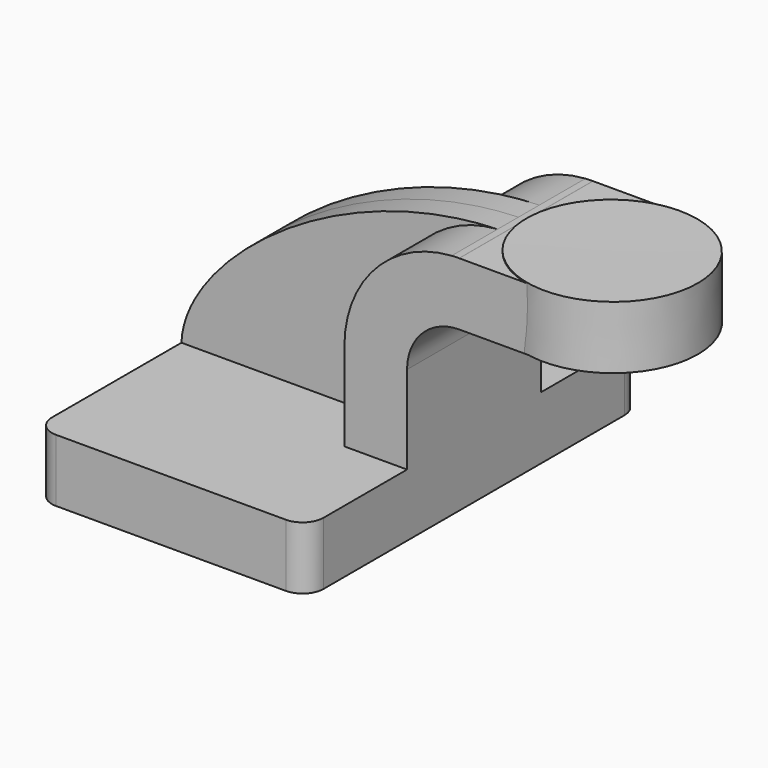
from build123d import *

# Parameters (mm, degrees)
F1_DEPTH = 63.5
F2_DEPTH = 25.4
F3_DEPTH = 7.9375
F5_R     = 6.35


# Not quite as in the source:
# - ends of sketch curves that miss each other by under 0.0002 mm in the source are joined


with BuildPart() as f1:
    # F0 (on Front) → F1 (new body, symmetric)
    with BuildSketch(Plane.XZ):
        Polygon((22.225, 9.525), (-41.275, 9.525), (-41.275, -9.525), (41.275, -9.525), (41.275, 9.525), align=None)
    extrude(amount=F1_DEPTH, both=True)

    # F0 (on Front) → F2 (join, symmetric)
    with BuildSketch(Plane.XZ):
        with BuildLine():
            Line((22.225, 36.2963777006), (22.225, 9.525))
            Line((22.225, 9.525), (41.275, 9.525))
            Line((41.275, 9.525), (41.275, 36.2963777006))
            ThreePointArc((41.275, 36.2963777006), (45.9064737786, 47.5034622059), (57.0984636988, 52.1712940471))
            Line((57.0984636988, 52.1712940471), (57.0984634272, 71.2213777006))
            ThreePointArc((57.0984634272, 71.2213777006), (55.9576218184, 71.2010172098), (54.8180528643, 71.1434385172))
            ThreePointArc((54.8180528643, 71.1434385172), (31.6431491682, 60.1533721811), (22.225, 36.2963777006))
        make_face()
        with BuildLine():
            ThreePointArc((57.15, 71.2213777006), (57.1242317347, 71.2213681944), (57.0984634834, 71.221339676))
            Line((57.0984634834, 71.221339676), (57.0984634272, 52.1713777006))
            ThreePointArc((57.0984634272, 52.1713777006), (57.1242318155, 52.1713567872), (57.15, 52.1713777006))
            Line((57.15, 52.1713777006), (83.1548832357, 52.1713777006))
            Line((83.1548832357, 52.1713777006), (83.2994319499, 71.2213777006))
            Line((83.2994319499, 71.2213777006), (57.15, 71.2213777006))
        make_face()
    extrude(amount=F2_DEPTH, both=True)

    # F0 (on Front) → F3 (join, symmetric)
    with BuildSketch(Plane.XZ):
        with BuildLine():
            add(Edge.make_bspline(
                [(-41.275, 9.525), (-40.4461435974, 33.376108855), (4.4869781457, 69.5420511852), (54.8180528643, 71.1434385172)],
                knots=[0, 0, 0, 0, 114.1521211983, 114.1521211983, 114.1521211983, 114.1521211983], degree=3))
            Line((-41.275, 9.525), (22.225, 9.525))
            Line((22.225, 9.525), (22.225, 36.2963777006))
            ThreePointArc((22.225, 36.2963777006), (31.6431491682, 60.1533721811), (54.8180528643, 71.1434385172))
        make_face()
    extrude(amount=F3_DEPTH, both=True)

    # F5
    f5_edges = [f1.edges().sort_by_distance(p)[0] for p in [
        (41.275, -63.5, 0),
        (-41.275, -63.5, 0),
        (41.275, 63.5, 0),
        (-41.275, 63.5, 0),
    ]]
    fillet(f5_edges, radius=F5_R)


with BuildPart() as f4:
    # F0 (on Front) → F4 (revolve)
    with BuildSketch(Plane.XZ):
        Polygon((109.3558517583, 71.2213777006), (83.2994319499, 71.2213777006), (83.1548832357, 52.1713777006), (109.3558517583, 52.1713777006), align=None)
    revolve(axis=Axis((83.2271575928, 0, 61.6963777006), (-0.0075876406, 0, -0.9999712134)))


solid = Compound([f1.part, f4.part])
